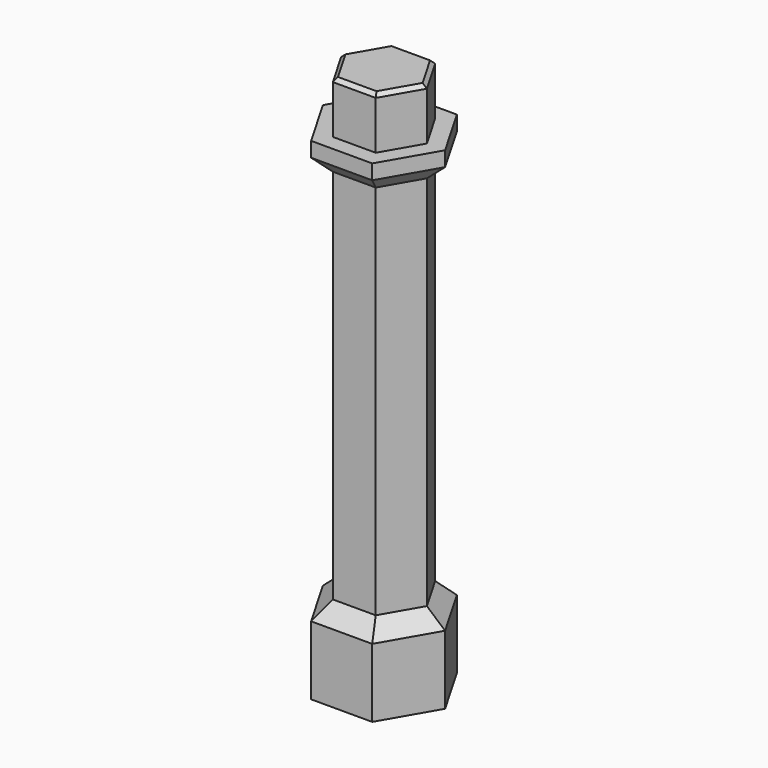
from build123d import *

# Parameters (mm, degrees)
F1_DEPTH = 65.95
F3_DEPTH = 7.25
F5_DEPTH = 2
F8_DEPTH = 2
F9_SIZE  = 0.5
F10_SIZE = 2.12499


# Not quite as in the source:
# - a fillet or chamfer is up to 0.001 mm smaller than in the source, because OpenCascade refuses the exact size


with BuildPart() as f1:
    # F0 (on Top) → F1 (new body)
    with BuildSketch(Plane.XY):
        Polygon((-2.8867513459, -5), (2.8867513459, -5), (5.7735026919, 0), (2.8867513459, 5), (-2.8867513459, 5), (-5.7735026919, 0), align=None)
    extrude(amount=-F1_DEPTH)



with BuildPart() as f3:
    # F2 (on face) → F3 (new body)
    with BuildSketch(Plane(origin=(0, 0, -65.95), x_dir=(1, 0, 0), z_dir=(0, 0, -1))):
        Polygon((4.113620668, 7.125), (-4.113620668, 7.125), (-8.227241336, 0), (-4.113620668, -7.125), (4.113620668, -7.125), (8.227241336, 0), align=None)
        Polygon((2.9589201296, 5.125), (5.9178402592, 0), (2.9589201296, -5.125), (-2.9589201296, -5.125), (-5.9178402592, 0), (-2.9589201296, 5.125), align=None, mode=Mode.SUBTRACT)
    extrude(amount=F3_DEPTH)


with BuildPart() as f1_1:
    add(f1.part)

    add(f3.part)  # F5 merges F3
    # F4 (on face) → F5 (join)
    with BuildSketch(Plane.XY.offset(-65.95)):
        Polygon((-8.227241336, 0), (-4.113620668, -7.125), (4.113620668, -7.125), (8.227241336, 0), (4.113620668, 7.125), (-4.113620668, 7.125), align=None)
    extrude(amount=F5_DEPTH)

    # F7 (on offset) → F8 (join)
    with BuildSketch(Plane.XY.offset(-7)):
        Polygon((-8.227241336, 0), (-4.113620668, -7.125), (4.113620668, -7.125), (8.227241336, 0), (4.113620668, 7.125), (-4.113620668, 7.125), align=None)
    extrude(amount=-F8_DEPTH)

    # F9
    f9_edges = [f1_1.edges().sort_by_distance(p)[0] for p in [
        (-4.330127, -2.5, 0),
        (0, -5, 0),
        (4.330127, -2.5, 0),
        (4.330127, 2.5, 0),
        (0, 5, 0),
        (-4.330127, 2.5, 0),
        (-4.43838, 2.5625, -73.2),
        (-4.43838, -2.5625, -73.2),
        (0, -5.125, -73.2),
        (4.43838, -2.5625, -73.2),
        (4.43838, 2.5625, -73.2),
        (0, 5.125, -73.2),
    ]]
    chamfer(f9_edges, length=F9_SIZE)

    # F10 (size 2.125 in the source; OpenCascade refuses exactly that, so slightly less here)
    f10_edges = [f1_1.edges().sort_by_distance(p)[0] for p in [
        (0, 5, -63.95),
        (-4.330127, 2.5, -63.95),
        (-4.330127, -2.5, -63.95),
        (0, -5, -63.95),
        (4.330127, -2.5, -63.95),
        (4.330127, 2.5, -63.95),
        (-4.330127, 2.5, -9),
        (0, 5, -9),
        (-4.330127, -2.5, -9),
        (0, -5, -9),
        (4.330127, -2.5, -9),
        (4.330127, 2.5, -9),
    ]]
    chamfer(f10_edges, length=F10_SIZE)


solid = f1_1.part
